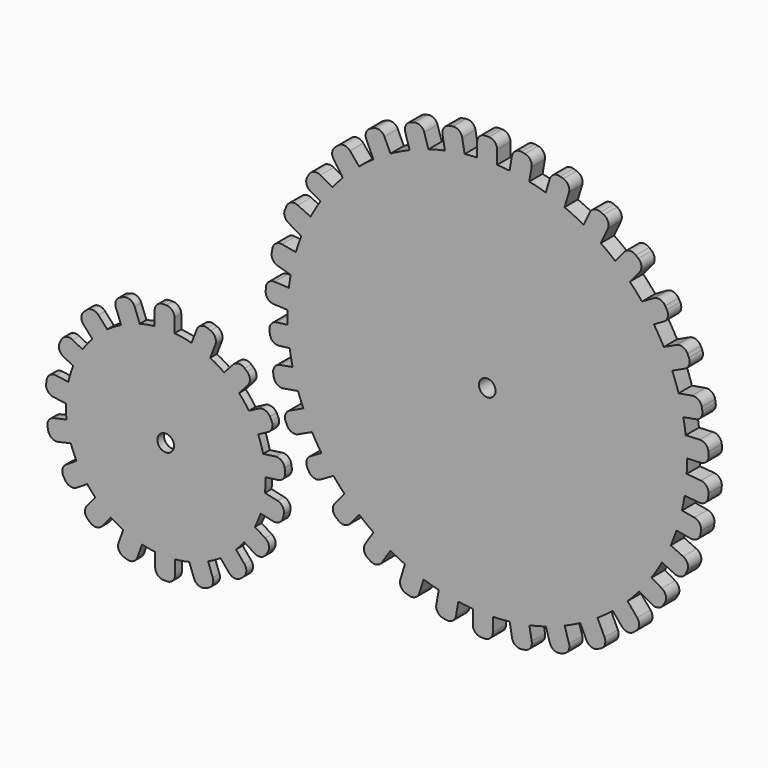
from build123d import *

# Parameters (mm, degrees)
F0_R     = 152.4
F0_R_2   = 6.35
F1_DEPTH = 12.7
F2_DEPTH = 6.35
F0_R_3   = 76.2
F4_DEPTH = 6.35
F6_DEPTH = 12.7


# Not quite as in the source:
# - a feature names something its author has since deleted; it is built from what else it names


with BuildPart() as f1:
    # F0 (on Front) → F1 (new body)
    with BuildSketch(Plane.XZ):
        with Locations((106.3798104379, 71.6841260691)):
            Circle(F0_R)
        with Locations((106.3798104379, 71.6841260691)):
            Circle(F0_R_2, mode=Mode.SUBTRACT)
    extrude(amount=F1_DEPTH)



with BuildPart() as f2:
    # F0 (on Front) → F2 (new body)
    with BuildSketch(Plane.XZ):
        with Locations((106.3798104379, 71.6841260691)):
            Circle(F0_R)
        with Locations((106.3798104379, 71.6841260691)):
            Circle(F0_R_2, mode=Mode.SUBTRACT)
    extrude(amount=F2_DEPTH)


with BuildPart() as f2b:
    # F0 (on Front) → F2, piece 2 (new body)
    with BuildSketch(Plane.XZ):
        with Locations((-144.0049031971, -49.3225429525)):
            Circle(F0_R_3)
        with Locations((-144.0049031971, -49.3225429525)):
            Circle(F0_R_2, mode=Mode.SUBTRACT)
    extrude(amount=F2_DEPTH)

    # F3 (on Front) → F4 (join)
    with BuildSketch(Plane.XZ):
        with BuildLine():
            Line((-204.3541227961, 20.4043868609), (-206.2390357075, 18.7018289862))
            ThreePointArc((-206.2390357075, 18.7018289862), (-208.3244533212, 14.3119079154), (-206.6949232994, 9.7331520212))
            Line((-206.6949232994, 9.7331520212), (-197.7369862783, -0.1842383959))
            ThreePointArc((-197.7369862783, -0.1842383959), (-197.2368223063, 0.0633153872), (-196.7901747778, 0.3979089611))
            Line((-196.7901747778, 0.3979089611), (-186.8162867746, 9.4068777351))
            ThreePointArc((-186.8162867746, 9.4068777351), (-186.5669051491, 9.6622880356), (-186.3514432182, 9.9468961399))
            Line((-186.3514432182, 9.9468961399), (-195.385445831, 19.948499269))
            ThreePointArc((-195.385445831, 19.948499269), (-199.7753669018, 22.0339168827), (-204.3541227961, 20.4043868609))
        make_face()
        with BuildLine():
            Line((-175.9440643065, 38.2304394299), (-178.3166684336, 37.3236044635))
            ThreePointArc((-178.3166684336, 37.3236044635), (-181.8468650713, 33.9832324288), (-181.9810913353, 29.1250067299))
            Line((-181.9810913353, 29.1250067299), (-176.9224404874, 15.8897695325))
            ThreePointArc((-176.9224404874, 15.8897695325), (-176.1952999555, 15.8943770065), (-175.4899473838, 16.0711037211))
            Line((-175.4899473838, 16.0711037211), (-164.0824814241, 20.4311606274))
            ThreePointArc((-164.0824814241, 20.4311606274), (-163.3354211249, 20.8437992565), (-162.7309690679, 21.446300244))
            Line((-162.7309690679, 21.446300244), (-167.7454665729, 34.5660165282))
            ThreePointArc((-167.7454665729, 34.5660165282), (-171.0858386076, 38.0962131659), (-175.9440643065, 38.2304394299))
        make_face()
        with BuildLine():
            Line((-143.5588021765, 43.2886108524), (-146.0988021765, 43.2886108524))
            ThreePointArc((-146.0988021765, 43.2886108524), (-150.588930237, 41.4287389129), (-152.4488021765, 36.9386108524))
            Line((-152.4488021765, 36.9386108524), (-152.4488021765, 23.5057070002))
            ThreePointArc((-152.4488021765, 23.5057070002), (-151.6256232188, 23.1059804274), (-150.7208942376, 22.9686108524))
            Line((-150.7208942376, 22.9686108524), (-138.5009451281, 22.9686108524))
            ThreePointArc((-138.5009451281, 22.9686108524), (-137.839627668, 23.0400251748), (-137.2088021765, 23.2509753769))
            Line((-137.2088021765, 23.2509753769), (-137.2088021765, 36.9386108524))
            ThreePointArc((-137.2088021765, 36.9386108524), (-139.068674116, 41.4287389129), (-143.5588021765, 43.2886108524))
        make_face()
        with BuildLine():
            ThreePointArc((-136.7876924353, -121.9389588268), (-137.3979774133, -121.7366523901), (-138.0371213199, -121.6668618795))
            Line((-138.0371213199, -121.6668618795), (-150.2997844964, -121.6668618795))
            ThreePointArc((-150.2997844964, -121.6668618795), (-151.2045134775, -121.8042314545), (-152.0276924353, -122.2039580274))
            Line((-152.0276924353, -122.2039580274), (-152.0276924353, -135.6368618795))
            ThreePointArc((-152.0276924353, -135.6368618795), (-150.1678204958, -140.12698994), (-145.6776924353, -141.9868618795))
            Line((-145.6776924353, -141.9868618795), (-143.1376924353, -141.9868618795))
            ThreePointArc((-143.1376924353, -141.9868618795), (-138.6475643747, -140.12698994), (-136.7876924353, -135.6368618795))
            Line((-136.7876924353, -135.6368618795), (-136.7876924353, -121.9389588268))
        make_face()
        with BuildLine():
            Line((-176.1923408536, -136.209608787), (-173.8052031826, -137.0774646159))
            ThreePointArc((-173.8052031826, -137.0774646159), (-168.9498273777, -136.8636903798), (-165.6677194328, -133.2792600109))
            Line((-165.6677194328, -133.2792600109), (-161.0693512083, -120.6309172247))
            ThreePointArc((-161.0693512083, -120.6309172247), (-161.7072488958, -119.9716351287), (-162.5124216468, -119.5320180423))
            Line((-162.5124216468, -119.5320180423), (-174.0098497748, -115.352070593))
            ThreePointArc((-174.0098497748, -115.352070593), (-174.6466853985, -115.1950207291), (-175.3023439103, -115.1766853205))
            Line((-175.3023439103, -115.1766853205), (-179.9905454586, -128.0721250372))
            ThreePointArc((-179.9905454586, -128.0721250372), (-179.7767712225, -132.9275008421), (-176.1923408536, -136.209608787))
        make_face()
        with BuildLine():
            Line((-203.3549844428, -120.0477373129), (-201.4090389886, -121.6801883196))
            ThreePointArc((-201.4090389886, -121.6801883196), (-196.7737263477, -123.1410956924), (-192.4630478364, -120.896452201))
            Line((-192.4630478364, -120.896452201), (-183.9812839196, -110.7858578437))
            ThreePointArc((-183.9812839196, -110.7858578437), (-184.3549387066, -109.9422037243), (-184.9639288475, -109.249021799))
            Line((-184.9639288475, -109.249021799), (-194.2361061545, -101.4706048106))
            ThreePointArc((-194.2361061545, -101.4706048106), (-194.8375854554, -101.0724913905), (-195.513143576, -100.8197210002))
            Line((-195.513143576, -100.8197210002), (-204.1387205614, -111.1017461607))
            ThreePointArc((-204.1387205614, -111.1017461607), (-205.5996279342, -115.7370588016), (-203.3549844428, -120.0477373129))
        make_face()
        with BuildLine():
            Line((-221.9770111308, -97.3072408044), (-220.6216536657, -99.455404239))
            ThreePointArc((-220.6216536657, -99.455404239), (-216.6527412723, -102.2604190419), (-211.8628514165, -101.437419163))
            Line((-211.8628514165, -101.437419163), (-201.5058619351, -94.902803229))
            ThreePointArc((-201.5058619351, -94.902803229), (-201.5923544651, -93.9512185842), (-201.9692402688, -93.0731802109))
            Line((-201.9692402688, -93.0731802109), (-208.5151537797, -82.6982847217))
            ThreePointArc((-208.5151537797, -82.6982847217), (-208.8884745428, -82.2224930782), (-209.3507880128, -81.8326054847))
            Line((-209.3507880128, -81.8326054847), (-219.9949962067, -88.5484385551))
            ThreePointArc((-219.9949962067, -88.5484385551), (-222.8000110096, -92.5173509486), (-221.9770111308, -97.3072408044))
        make_face()
        with BuildLine():
            Line((-234.1612291966, -67.9485382148), (-233.6126396119, -70.4285885101))
            ThreePointArc((-233.6126396119, -70.4285885101), (-230.8268862889, -74.4110440409), (-226.0410399119, -75.257240287))
            Line((-226.0410399119, -75.257240287), (-213.5840996431, -72.5017527468))
            ThreePointArc((-213.5840996431, -72.5017527468), (-213.3631563857, -71.6009829094), (-213.4233554896, -70.6754677605))
            Line((-213.4233554896, -70.6754677605), (-216.0944299344, -58.6001401358))
            ThreePointArc((-216.0944299344, -58.6001401358), (-216.2739099505, -58.0526065333), (-216.5576524317, -57.5511124393))
            Line((-216.5576524317, -57.5511124393), (-229.3325774197, -60.3769385147))
            ThreePointArc((-229.3325774197, -60.3769385147), (-233.3150329505, -63.1626918378), (-234.1612291966, -67.9485382148))
        make_face()
        with BuildLine():
            Line((-234.8751289908, -36.6048873101), (-235.2255460205, -39.1205995164))
            ThreePointArc((-235.2255460205, -39.1205995164), (-234.002914051, -43.8243793474), (-229.8123080788, -46.2859226067))
            Line((-229.8123080788, -46.2859226067), (-217.3849709244, -48.0169435724))
            ThreePointArc((-217.3849709244, -48.0169435724), (-216.82360206, -47.2265512804), (-216.5388459922, -46.2998534014))
            Line((-216.5388459922, -46.2998534014), (-214.8767964914, -34.3676758463))
            ThreePointArc((-214.8767964914, -34.3676758463), (-214.85853174, -33.6579630312), (-214.9993070039, -32.9621123245))
            Line((-214.9993070039, -32.9621123245), (-227.7098059006, -31.1916493684))
            ThreePointArc((-227.7098059006, -31.1916493684), (-232.4135857316, -32.4142813379), (-234.8751289908, -36.6048873101))
        make_face()
        with BuildLine():
            Line((-223.6030855792, -5.7841174114), (-224.7931154321, -8.0280935586))
            ThreePointArc((-224.7931154321, -8.0280935586), (-225.2536973874, -12.8662996202), (-222.1582496963, -16.6131085589))
            Line((-222.1582496963, -16.6131085589), (-212.1649924882, -21.9127524166))
            ThreePointArc((-212.1649924882, -21.9127524166), (-211.3178403266, -21.3555585105), (-210.7003788408, -20.5512742651))
            Line((-210.7003788408, -20.5512742651), (-204.9780904375, -9.7610586642))
            ThreePointArc((-204.9780904375, -9.7610586642), (-204.7580002749, -9.2207880669), (-204.6505108486, -8.6473963847))
            Line((-204.6505108486, -8.6473963847), (-215.0180705789, -3.1492516757))
            ThreePointArc((-215.0180705789, -3.1492516757), (-219.8562766405, -2.6886697204), (-223.6030855792, -5.7841174114))
        make_face()
        with BuildLine():
            Line((-114.0931942582, -115.352070593), (-125.5906223862, -119.5320180423))
            ThreePointArc((-125.5906223862, -119.5320180423), (-126.3957951373, -119.9716351287), (-127.0336928247, -120.6309172247))
            Line((-127.0336928247, -120.6309172247), (-122.4353246002, -133.2792600109))
            ThreePointArc((-122.4353246002, -133.2792600109), (-119.1532166553, -136.8636903798), (-114.2978408504, -137.0774646159))
            Line((-114.2978408504, -137.0774646159), (-111.9107031794, -136.209608787))
            ThreePointArc((-111.9107031794, -136.209608787), (-108.3262728106, -132.9275008421), (-108.1124985744, -128.0721250372))
            Line((-108.1124985744, -128.0721250372), (-112.8007001228, -115.1766853205))
            ThreePointArc((-112.8007001228, -115.1766853205), (-113.4563586346, -115.1950207291), (-114.0931942582, -115.352070593))
        make_face()
        with BuildLine():
            Line((-93.8669378785, -101.4706048106), (-103.1391151855, -109.249021799))
            ThreePointArc((-103.1391151855, -109.249021799), (-103.7481053264, -109.9422037243), (-104.1217601134, -110.7858578437))
            Line((-104.1217601134, -110.7858578437), (-95.6399961967, -120.896452201))
            ThreePointArc((-95.6399961967, -120.896452201), (-91.3293176854, -123.1410956924), (-86.6940050444, -121.6801883196))
            Line((-86.6940050444, -121.6801883196), (-84.7480595902, -120.0477373129))
            ThreePointArc((-84.7480595902, -120.0477373129), (-82.5034160989, -115.7370588016), (-83.9643234716, -111.1017461607))
            Line((-83.9643234716, -111.1017461607), (-92.589900457, -100.8197210002))
            ThreePointArc((-92.589900457, -100.8197210002), (-93.2654585777, -101.0724913905), (-93.8669378785, -101.4706048106))
        make_face()
        with BuildLine():
            Line((-79.5878902534, -82.6982847217), (-86.1338037642, -93.0731802109))
            ThreePointArc((-86.1338037642, -93.0731802109), (-86.5106895679, -93.9512185842), (-86.5971820979, -94.902803229))
            Line((-86.5971820979, -94.902803229), (-76.2401926166, -101.437419163))
            ThreePointArc((-76.2401926166, -101.437419163), (-71.4503027608, -102.2604190419), (-67.4813903673, -99.455404239))
            Line((-67.4813903673, -99.455404239), (-66.1260329023, -97.3072408044))
            ThreePointArc((-66.1260329023, -97.3072408044), (-65.3030330234, -92.5173509486), (-68.1080478263, -88.5484385551))
            Line((-68.1080478263, -88.5484385551), (-78.7522560203, -81.8326054847))
            ThreePointArc((-78.7522560203, -81.8326054847), (-79.2145694903, -82.2224930782), (-79.5878902534, -82.6982847217))
        make_face()
        with BuildLine():
            ThreePointArc((-71.5453916014, -57.5511124393), (-71.8291340826, -58.0526065333), (-72.0086140986, -58.6001401358))
            Line((-72.0086140986, -58.6001401358), (-74.6796885435, -70.6754677605))
            ThreePointArc((-74.6796885435, -70.6754677605), (-74.7398876473, -71.6009829094), (-74.51894439, -72.5017527468))
            Line((-74.51894439, -72.5017527468), (-62.0620041212, -75.257240287))
            ThreePointArc((-62.0620041212, -75.257240287), (-57.2761577442, -74.4110440409), (-54.4904044211, -70.4285885101))
            Line((-54.4904044211, -70.4285885101), (-53.9418148365, -67.9485382148))
            ThreePointArc((-53.9418148365, -67.9485382148), (-54.7880110826, -63.1626918378), (-58.7704666133, -60.3769385147))
            Line((-58.7704666133, -60.3769385147), (-71.5453916014, -57.5511124393))
        make_face()
        with BuildLine():
            Line((-73.2262475416, -34.3676758463), (-71.5641980408, -46.2998534014))
            ThreePointArc((-71.5641980408, -46.2998534014), (-71.2794419731, -47.2265512804), (-70.7180731086, -48.0169435724))
            Line((-70.7180731086, -48.0169435724), (-58.2907359542, -46.2859226067))
            ThreePointArc((-58.2907359542, -46.2859226067), (-54.100129982, -43.8243793474), (-52.8774980126, -39.1205995164))
            Line((-52.8774980126, -39.1205995164), (-53.2279150423, -36.6048873101))
            ThreePointArc((-53.2279150423, -36.6048873101), (-55.6894583015, -32.4142813379), (-60.3932381325, -31.1916493684))
            Line((-60.3932381325, -31.1916493684), (-73.1037370291, -32.9621123245))
            ThreePointArc((-73.1037370291, -32.9621123245), (-73.2445122931, -33.6579630312), (-73.2262475416, -34.3676758463))
        make_face()
        with BuildLine():
            Line((-83.1249535955, -9.7610586642), (-77.4026651923, -20.5512742651))
            ThreePointArc((-77.4026651923, -20.5512742651), (-76.7852037064, -21.3555585105), (-75.9380515448, -21.9127524166))
            Line((-75.9380515448, -21.9127524166), (-65.9447943367, -16.6131085589))
            ThreePointArc((-65.9447943367, -16.6131085589), (-62.8493466457, -12.8662996202), (-63.309928601, -8.0280935586))
            Line((-63.309928601, -8.0280935586), (-64.4999584539, -5.7841174114))
            ThreePointArc((-64.4999584539, -5.7841174114), (-68.2467673926, -2.6886697204), (-73.0849734541, -3.1492516757))
            Line((-73.0849734541, -3.1492516757), (-83.4525331844, -8.6473963847))
            ThreePointArc((-83.4525331844, -8.6473963847), (-83.3450437581, -9.2207880669), (-83.1249535955, -9.7610586642))
        make_face()
        with BuildLine():
            ThreePointArc((-101.7516008148, 9.9468961399), (-101.5361388839, 9.6622880356), (-101.2867572584, 9.4068777351))
            Line((-101.2867572584, 9.4068777351), (-91.3128692552, 0.3979089611))
            ThreePointArc((-91.3128692552, 0.3979089611), (-90.8662217267, 0.0633153872), (-90.3660577547, -0.1842383959))
            Line((-90.3660577547, -0.1842383959), (-81.4081207337, 9.7331520212))
            ThreePointArc((-81.4081207337, 9.7331520212), (-79.7785907119, 14.3119079154), (-81.8640083256, 18.7018289862))
            Line((-81.8640083256, 18.7018289862), (-83.748921237, 20.4043868609))
            ThreePointArc((-83.748921237, 20.4043868609), (-88.3276771312, 22.0339168827), (-92.717598202, 19.948499269))
            Line((-92.717598202, 19.948499269), (-101.7516008148, 9.9468961399))
        make_face()
        with BuildLine():
            Line((-124.0205626089, 20.4311606274), (-112.6130966493, 16.0711037211))
            ThreePointArc((-112.6130966493, 16.0711037211), (-111.9077440776, 15.8943770065), (-111.1806035456, 15.8897695325))
            Line((-111.1806035456, 15.8897695325), (-106.1219526978, 29.1250067299))
            ThreePointArc((-106.1219526978, 29.1250067299), (-106.2561789618, 33.9832324288), (-109.7863755995, 37.3236044635))
            Line((-109.7863755995, 37.3236044635), (-112.1589797265, 38.2304394299))
            ThreePointArc((-112.1589797265, 38.2304394299), (-117.0172054254, 38.0962131659), (-120.3575774601, 34.5660165282))
            Line((-120.3575774601, 34.5660165282), (-125.3720749651, 21.446300244))
            ThreePointArc((-125.3720749651, 21.446300244), (-124.7676229082, 20.8437992565), (-124.0205626089, 20.4311606274))
        make_face()
    extrude(amount=F4_DEPTH)


with BuildPart() as f1_1:
    add(f1.part)

    add(f2.part)  # F6 merges F2
    # F5 (on Front) → F6 (join)
    with BuildSketch(Plane.XZ):
        with BuildLine():
            ThreePointArc((-1.0245592963, 176.3703184272), (-0.8688153261, 176.4703400406), (-0.7221504189, 176.5832555508))
            Line((-0.7221504189, 176.5832555508), (9.3414453239, 185.0377039154))
            ThreePointArc((9.3414453239, 185.0377039154), (9.9458045347, 185.7248391814), (10.3189656625, 186.5603963023))
            Line((10.3189656625, 186.5603963023), (1.6784122703, 196.8455187117))
            ThreePointArc((1.6784122703, 196.8455187117), (-2.6338498025, 199.0871184635), (-7.2681299416, 197.6229390948))
            Line((-7.2681299416, 197.6229390948), (-9.674904736, 195.6010024287))
            ThreePointArc((-9.674904736, 195.6010024287), (-11.6445782491, 192.6544180871), (-11.7281303758, 189.1111156624))
            Line((-11.7281303758, 189.1111156624), (-1.0245592963, 176.3703184272))
        make_face()
        with BuildLine():
            ThreePointArc((-3.9138862135, 177.021707564), (-2.5974272967, 176.1273439582), (-1.0245592963, 176.3703184272))
            Line((-1.0245592963, 176.3703184272), (-11.7281303758, 189.1111156624))
            ThreePointArc((-11.7281303758, 189.1111156624), (-11.3645228576, 188.0967954669), (-10.8346522218, 187.1585561608))
            Line((-10.8346522218, 187.1585561608), (-3.9138862135, 177.021707564))
        make_face()
        with BuildLine():
            ThreePointArc((47.8904068269, 209.8163499975), (48.12467512, 209.8475296096), (48.3540937879, 209.9042823727))
            Line((48.3540937879, 209.9042823727), (60.8237512144, 213.7288847809))
            ThreePointArc((60.8237512144, 213.7288847809), (61.6484290935, 214.1255096984), (62.3182107431, 214.7490459615))
            Line((62.3182107431, 214.7490459615), (58.3792777757, 227.5914644634))
            ThreePointArc((58.3792777757, 227.5914644634), (55.2845212205, 231.3388442807), (50.4464001936, 231.8003186148))
            Line((50.4464001936, 231.8003186148), (48.0180538469, 231.0555139287))
            ThreePointArc((48.0180538469, 231.0555139287), (44.2706740297, 227.9607573735), (43.8091996955, 223.1226363466))
            Line((43.8091996955, 223.1226363466), (47.8904068269, 209.8163499975))
        make_face()
        with BuildLine():
            Line((20.0982469166, 195.7489624087), (32.341001256, 201.4666191011))
            ThreePointArc((32.341001256, 201.4666191011), (33.1026111195, 201.9739211269), (33.6793151863, 202.6844261225))
            Line((33.6793151863, 202.6844261225), (27.9951670721, 214.8554312624))
            ThreePointArc((27.9951670721, 214.8554312624), (24.4100104736, 218.1367459068), (19.5546820949, 217.9218972006))
            Line((19.5546820949, 217.9218972006), (17.2532919118, 216.8470933928))
            ThreePointArc((17.2532919118, 216.8470933928), (13.9719772675, 213.2619367943), (14.1868259737, 208.4066084156))
            Line((14.1868259737, 208.4066084156), (20.0982469166, 195.7489624087))
        make_face()
        with BuildLine():
            Line((76.0232179502, 217.3823675227), (88.0025690396, 219.5019140519))
            ThreePointArc((88.0025690396, 219.5019140519), (88.8695271021, 219.7948110427), (89.6104726789, 220.3318441718))
            Line((89.6104726789, 220.3318441718), (87.2700951432, 233.5592981555))
            ThreePointArc((87.2700951432, 233.5592981555), (84.6563665163, 237.6567115221), (79.9108725033, 238.7058350626))
            Line((79.9108725033, 238.7058350626), (77.4097205939, 238.2632979161))
            ThreePointArc((77.4097205939, 238.2632979161), (73.3123072273, 235.6495692892), (72.2631836868, 230.9040752762))
            Line((72.2631836868, 230.9040752762), (74.6444925558, 217.4452836898))
            ThreePointArc((74.6444925558, 217.4452836898), (75.3303693298, 217.3374361651), (76.0232179502, 217.3823675227))
        make_face()
        with BuildLine():
            Line((260.2206908891, 142.0700291107), (259.1472405042, 144.3720508898))
            ThreePointArc((259.1472405042, 144.3720508898), (255.5640139667, 147.6554730697), (250.7085600945, 147.4434793754))
            Line((250.7085600945, 147.4434793754), (238.5342147308, 141.7664888993))
            ThreePointArc((238.5342147308, 141.7664888993), (238.5198298854, 140.8515036504), (238.7776857592, 139.9734858386))
            Line((238.7776857592, 139.9734858386), (243.9968427597, 128.7809675318))
            ThreePointArc((243.9968427597, 128.7809675318), (244.3021755744, 128.2686537818), (244.7042014135, 127.8281214551))
            Line((244.7042014135, 127.8281214551), (257.1492624034, 133.6313487009))
            ThreePointArc((257.1492624034, 133.6313487009), (260.4326845834, 137.2145752385), (260.2206908891, 142.0700291107))
        make_face()
        with BuildLine():
            Line((243.4403321706, 168.7168144661), (242.1771492341, 170.9204407658))
            ThreePointArc((242.1771492341, 170.9204407658), (238.3305681834, 173.8909942245), (233.5101261434, 173.2715491737))
            Line((233.5101261434, 173.2715491737), (221.8561496827, 166.5911495934))
            ThreePointArc((221.8561496827, 166.5911495934), (221.9187392987, 165.6781942443), (222.2494979612, 164.8249629528))
            Line((222.2494979612, 164.8249629528), (227.2753059104, 156.057426396))
            ThreePointArc((227.2753059104, 156.057426396), (228.5033787541, 154.6410178722), (230.1757037272, 153.7938430378))
            Line((230.1757037272, 153.7938430378), (241.0892237627, 160.0497913754))
            ThreePointArc((241.0892237627, 160.0497913754), (244.0597772214, 163.8963724261), (243.4403321706, 168.7168144661))
        make_face()
        with BuildLine():
            Line((275.2757229067, 81.0317905346), (275.1540238465, 83.568873375))
            ThreePointArc((275.1540238465, 83.568873375), (273.0811523708, 87.9647325033), (268.507069095, 89.6073328251))
            Line((268.507069095, 89.6073328251), (255.0895927725, 88.9637218899))
            ThreePointArc((255.0895927725, 88.9637218899), (254.7297662673, 88.1223362377), (254.6359027536, 87.2120645364))
            Line((254.6359027536, 87.2120645364), (255.223383884, 74.9647366469))
            ThreePointArc((255.223383884, 74.9647366469), (255.3229520685, 74.3287374111), (255.5557510616, 73.7285595374))
            Line((255.5557510616, 73.7285595374), (269.2372634566, 74.3848357831))
            ThreePointArc((269.2372634566, 74.3848357831), (273.633122585, 76.4577072588), (275.2757229067, 81.0317905346))
        make_face()
        with BuildLine():
            Line((-42.592206737, 75.5533938816), (-42.0119272421, 87.8010650977))
            ThreePointArc((-42.0119272421, 87.8010650977), (-42.1063259871, 88.7112814492), (-42.4666471721, 89.5524553748))
            Line((-42.4666471721, 89.5524553748), (-55.8844996237, 90.1881766076))
            ThreePointArc((-55.8844996237, 90.1881766076), (-60.4576162457, 88.5428869696), (-62.5279025602, 84.1458097349))
            Line((-62.5279025602, 84.1458097349), (-62.6481097729, 81.6086557731))
            ThreePointArc((-62.6481097729, 81.6086557731), (-61.0028201349, 77.0355391511), (-56.6057429003, 74.9652528367))
            Line((-56.6057429003, 74.9652528367), (-42.9238469745, 74.3170215511))
            ThreePointArc((-42.9238469745, 74.3170215511), (-42.6914009313, 74.9173362088), (-42.592206737, 75.5533938816))
        make_face()
        with BuildLine():
            Line((270.5131564686, 109.6682831591), (270.0720900973, 112.1696948517))
            ThreePointArc((270.0720900973, 112.1696948517), (267.4607712365, 116.2686444048), (262.7158949375, 117.3205581552))
            Line((262.7158949375, 117.3205581552), (249.4870670785, 114.9879588805))
            ThreePointArc((249.4870670785, 114.9879588805), (249.2363567764, 114.1078740698), (249.2581786927, 113.1930359784))
            Line((249.2581786927, 113.1930359784), (251.2121747594, 102.1113736095))
            ThreePointArc((251.2121747594, 102.1113736095), (251.5913543929, 100.9785648168), (252.2853940364, 100.0062778589))
            Line((252.2853940364, 100.0062778589), (265.3622931652, 102.3120879993))
            ThreePointArc((265.3622931652, 102.3120879993), (269.4612427182, 104.9234068601), (270.5131564686, 109.6682831591))
        make_face()
        with BuildLine():
            Line((-38.6289994987, 102.0261590536), (-36.6815198823, 113.1089684732))
            ThreePointArc((-36.6815198823, 113.1089684732), (-36.6602359024, 114.0238192379), (-36.9114636586, 114.9037564765))
            Line((-36.9114636586, 114.9037564765), (-50.1416608191, 117.2285766837))
            ThreePointArc((-50.1416608191, 117.2285766837), (-54.8859177635, 116.1738730872), (-57.4948259553, 112.0733887649))
            Line((-57.4948259553, 112.0733887649), (-58.0494006059, 108.9173890257))
            ThreePointArc((-58.0494006059, 108.9173890257), (-57.6906086949, 105.4589639964), (-55.564270848, 102.707941881))
            Line((-55.564270848, 102.707941881), (-39.7009807757, 99.9204326047))
            ThreePointArc((-39.7009807757, 99.9204326047), (-39.0075129654, 100.8931274958), (-38.6289994987, 102.0261590536))
        make_face()
        with BuildLine():
            Line((-31.4293506964, 128.6999910423), (-26.2167758949, 139.8955763233))
            ThreePointArc((-26.2167758949, 139.8955763233), (-25.9594363477, 140.7737456048), (-25.9743592098, 141.6887222371))
            Line((-25.9743592098, 141.6887222371), (-38.152040588, 147.3585531123))
            ThreePointArc((-38.152040588, 147.3585531123), (-43.0076182748, 147.5676917214), (-46.5889135125, 144.2821631411))
            Line((-46.5889135125, 144.2821631411), (-47.9254367671, 141.4115741048))
            ThreePointArc((-47.9254367671, 141.4115741048), (-48.46871671, 137.9353323342), (-47.0778609789, 134.7034705984))
            Line((-47.0778609789, 134.7034705984), (-32.1361489462, 127.7467291975))
            ThreePointArc((-32.1361489462, 127.7467291975), (-31.7343822134, 128.1874978426), (-31.4293506964, 128.6999910423))
        make_face()
        with BuildLine():
            Line((-59.7967524833, 56.3136117376), (-59.4702737563, 53.7946810834))
            ThreePointArc((-59.4702737563, 53.7946810834), (-57.0486911835, 49.5808572292), (-52.3567503031, 48.3135512655))
            Line((-52.3567503031, 48.3135512655), (-41.8407955625, 49.6765246811))
            ThreePointArc((-41.8407955625, 49.6765246811), (-41.3847741945, 50.6920760446), (-41.3238471288, 51.8036460841))
            Line((-41.3238471288, 51.8036460841), (-43.0201186457, 64.8911460272))
            Line((-43.0201186457, 64.8911460272), (-54.3156226654, 63.4271351908))
            ThreePointArc((-54.3156226654, 63.4271351908), (-58.5294465197, 61.0055526181), (-59.7967524833, 56.3136117376))
        make_face()
        with BuildLine():
            Line((274.9560192353, 53.0251019398), (275.1773948219, 55.555436473))
            ThreePointArc((275.1773948219, 55.555436473), (273.7159407028, 60.190576761), (269.4049974554, 62.4347117723))
            Line((269.4049974554, 62.4347117723), (255.9048884791, 63.6158182641))
            ThreePointArc((255.9048884791, 63.6158182641), (255.4396240069, 62.8338566279), (255.2259104079, 61.9494011302))
            Line((255.2259104079, 61.9494011302), (254.3361911927, 51.7798639654))
            ThreePointArc((254.3361911927, 51.7798639654), (255.0985326357, 49.3620258071), (257.3472591972, 48.1914128535))
            Line((257.3472591972, 48.1914128535), (268.076743936, 47.2527045734))
            ThreePointArc((268.076743936, 47.2527045734), (272.7118842239, 48.7141586925), (274.9560192353, 53.0251019398))
        make_face()
        with BuildLine():
            Line((-14.7238555296, 155.9862775982), (-9.7032038361, 164.7567678576))
            ThreePointArc((-9.7032038361, 164.7567678576), (-9.372946938, 165.6101934904), (-9.3108941585, 166.5231854849))
            Line((-9.3108941585, 166.5231854849), (-20.9687967367, 173.1967312723))
            ThreePointArc((-20.9687967367, 173.1967312723), (-25.7896021823, 173.8133417547), (-29.6344358572, 170.8405269868))
            Line((-29.6344358572, 170.8405269868), (-30.8963228241, 168.6361583056))
            ThreePointArc((-30.8963228241, 168.6361583056), (-31.5129333066, 163.8153528601), (-28.5401185387, 159.9705191852))
            Line((-28.5401185387, 159.9705191852), (-17.6229218386, 153.7209891726))
            ThreePointArc((-17.6229218386, 153.7209891726), (-15.9510953007, 154.5691472019), (-14.7238555296, 155.9862775982))
        make_face()
        with BuildLine():
            ThreePointArc((-35.6241415015, 127.4124404853), (-33.8252209145, 127.0065006326), (-32.1361489462, 127.7467291975))
            Line((-32.1361489462, 127.7467291975), (-47.0778609789, 134.7034705984))
            ThreePointArc((-47.0778609789, 134.7034705984), (-46.3154336955, 133.9221774935), (-45.4304545802, 133.283016916))
            Line((-45.4304545802, 133.283016916), (-35.6241415015, 127.4124404853))
        make_face()
        with BuildLine():
            ThreePointArc((-43.7381548127, 98.8491770261), (-41.5702894989, 98.822229021), (-39.7009807757, 99.9204326047))
            Line((-39.7009807757, 99.9204326047), (-55.564270848, 102.707941881))
            ThreePointArc((-55.564270848, 102.707941881), (-54.6134250826, 102.1280363601), (-53.575886004, 101.7231774427))
            Line((-53.575886004, 101.7231774427), (-43.7381548127, 98.8491770261))
        make_face()
        with BuildLine():
            Line((251.6045288556, 99.8862229573), (252.2853940364, 100.0062778589))
            ThreePointArc((252.2853940364, 100.0062778589), (251.5913543929, 100.9785648168), (251.2121747594, 102.1113736095))
            Line((251.2121747594, 102.1113736095), (251.6045288556, 99.8862229573))
        make_face()
        with BuildLine():
            Line((-16.4160907922, 153.0301408668), (-14.7238555296, 155.9862775982))
            ThreePointArc((-14.7238555296, 155.9862775982), (-15.9510953007, 154.5691472019), (-17.6229218386, 153.7209891726))
            Line((-17.6229218386, 153.7209891726), (-16.4160907922, 153.0301408668))
        make_face()
        with BuildLine():
            ThreePointArc((203.1929267292, 185.0946970875), (202.5881635814, 185.7814768663), (202.2145112034, 186.6168144208))
            Line((202.2145112034, 186.6168144208), (201.8692724544, 186.2053749013))
            Line((201.8692724544, 186.2053749013), (203.1929267292, 185.0946970875))
        make_face()
        with BuildLine():
            ThreePointArc((10.3189656625, 186.5603963023), (9.9458045347, 185.7248391814), (9.3414453239, 185.0377039154))
            Line((9.3414453239, 185.0377039154), (10.6644462818, 186.1491598573))
            Line((10.6644462818, 186.1491598573), (10.3189656625, 186.5603963023))
        make_face()
        with BuildLine():
            Line((228.9692791142, 153.1022852244), (230.1757037272, 153.7938430378))
            ThreePointArc((230.1757037272, 153.7938430378), (228.5033787541, 154.6410178722), (227.2753059104, 156.057426396))
            Line((227.2753059104, 156.057426396), (228.9692791142, 153.1022852244))
        make_face()
        with BuildLine():
            Line((-42.0119272421, 87.8010650977), (-41.9301528337, 89.5270369375))
            Line((-41.9301528337, 89.5270369375), (-42.4666471721, 89.5524553748))
            ThreePointArc((-42.4666471721, 89.5524553748), (-42.1063259871, 88.7112814492), (-42.0119272421, 87.8010650977))
        make_face()
        with BuildLine():
            ThreePointArc((-41.3238471288, 51.8036460841), (-41.3847741945, 50.6920760446), (-41.8407955625, 49.6765246811))
            Line((-41.8407955625, 49.6765246811), (-41.0612462834, 49.7775621019))
            Line((-41.0612462834, 49.7775621019), (-41.3238471288, 51.8036460841))
        make_face()
        with BuildLine():
            Line((254.047499639, 48.4801044072), (257.3472591972, 48.1914128535))
            ThreePointArc((257.3472591972, 48.1914128535), (255.0985326357, 49.3620258071), (254.3361911927, 51.7798639654))
            Line((254.3361911927, 51.7798639654), (254.047499639, 48.4801044072))
        make_face()
        with BuildLine():
            Line((-39.0200451193, 99.8007780784), (-38.6289994987, 102.0261590536))
            ThreePointArc((-38.6289994987, 102.0261590536), (-39.0075129654, 100.8931274958), (-39.7009807757, 99.9204326047))
            Line((-39.7009807757, 99.9204326047), (-39.0200451193, 99.8007780784))
        make_face()
        with BuildLine():
            Line((-36.6815198823, 113.1089684732), (-36.3824724584, 114.8108017445))
            Line((-36.3824724584, 114.8108017445), (-36.9114636586, 114.9037564765))
            ThreePointArc((-36.9114636586, 114.9037564765), (-36.6602359024, 114.0238192379), (-36.6815198823, 113.1089684732))
        make_face()
        with BuildLine():
            Line((-26.2167758949, 139.8955763233), (-25.4874514027, 141.4620218635))
            Line((-25.4874514027, 141.4620218635), (-25.9743592098, 141.6887222371))
            ThreePointArc((-25.9743592098, 141.6887222371), (-25.9594363477, 140.7737456048), (-26.2167758949, 139.8955763233))
        make_face()
        with BuildLine():
            Line((-42.6513961102, 74.3041131665), (-42.592206737, 75.5533938816))
            ThreePointArc((-42.592206737, 75.5533938816), (-42.6914009313, 74.9173362088), (-42.9238469745, 74.3170215511))
            Line((-42.9238469745, 74.3170215511), (-42.6513961102, 74.3041131665))
        make_face()
        with BuildLine():
            ThreePointArc((249.2581786927, 113.1930359784), (249.2363567764, 114.1078740698), (249.4870670785, 114.9879588805))
            Line((249.4870670785, 114.9879588805), (248.9581306279, 114.8946931132))
            Line((248.9581306279, 114.8946931132), (249.2581786927, 113.1930359784))
        make_face()
        with BuildLine():
            ThreePointArc((255.2259104079, 61.9494011302), (255.4396240069, 62.8338566279), (255.9048884791, 63.6158182641))
            Line((255.9048884791, 63.6158182641), (255.3757531585, 63.6621116061))
            Line((255.3757531585, 63.6621116061), (255.2259104079, 61.9494011302))
        make_face()
        with BuildLine():
            ThreePointArc((254.6359027536, 87.2120645364), (254.7297662673, 88.1223362377), (255.0895927725, 88.9637218899))
            Line((255.0895927725, 88.9637218899), (254.5531134731, 88.9379879936))
            Line((254.5531134731, 88.9379879936), (254.6359027536, 87.2120645364))
        make_face()
        with BuildLine():
            ThreePointArc((222.2494979612, 164.8249629528), (221.9187392987, 165.6781942443), (221.8561496827, 166.5911495934))
            Line((221.8561496827, 166.5911495934), (221.3901814949, 166.3240430228))
            Line((221.3901814949, 166.3240430228), (222.2494979612, 164.8249629528))
        make_face()
        with BuildLine():
            Line((-9.7032038361, 164.7567678576), (-8.8447689903, 166.2563529538))
            Line((-8.8447689903, 166.2563529538), (-9.3108941585, 166.5231854849))
            ThreePointArc((-9.3108941585, 166.5231854849), (-9.372946938, 165.6101934904), (-9.7032038361, 164.7567678576))
        make_face()
        with BuildLine():
            ThreePointArc((238.7776857592, 139.9734858386), (238.5198298854, 140.8515036504), (238.5342147308, 141.7664888993))
            Line((238.5342147308, 141.7664888993), (238.0474403096, 141.5395022589))
            Line((238.0474403096, 141.5395022589), (238.7776857592, 139.9734858386))
        make_face()
        with BuildLine():
            Line((-31.9200309468, 127.6461063886), (-31.4293506964, 128.6999910423))
            ThreePointArc((-31.4293506964, 128.6999910423), (-31.7343822134, 128.1874978426), (-32.1361489462, 127.7467291975))
            Line((-32.1361489462, 127.7467291975), (-31.9200309468, 127.6461063886))
        make_face()
        with BuildLine():
            Line((255.2833078347, 73.7154909516), (255.5557510616, 73.7285595374))
            ThreePointArc((255.5557510616, 73.7285595374), (255.3229520685, 74.3287374111), (255.223383884, 74.9647366469))
            Line((255.223383884, 74.9647366469), (255.2833078347, 73.7154909516))
        make_face()
        with BuildLine():
            Line((213.5437897675, 176.4092917297), (213.5640260545, 176.4334083973))
            ThreePointArc((213.5640260545, 176.4334083973), (213.4082232976, 176.5333384147), (213.2614920205, 176.6461676651))
            Line((213.2614920205, 176.6461676651), (213.5437897675, 176.4092917297))
        make_face()
        with BuildLine():
            Line((-1.0245592963, 176.3703184272), (-1.0043088321, 176.3462136628))
            Line((-1.0043088321, 176.3462136628), (-0.7221504189, 176.5832555508))
            ThreePointArc((-0.7221504189, 176.5832555508), (-0.8688153261, 176.4703400406), (-1.0245592963, 176.3703184272))
        make_face()
        with BuildLine():
            Line((244.4881426185, 127.7273715844), (244.7042014135, 127.8281214551))
            ThreePointArc((244.7042014135, 127.8281214551), (244.3021755744, 128.2686537818), (243.9968427597, 128.7809675318))
            Line((243.9968427597, 128.7809675318), (244.4881426185, 127.7273715844))
        make_face()
        with BuildLine():
            Line((195.2623773151, 216.8994288321), (192.9603555361, 217.9728792169))
            ThreePointArc((192.9603555361, 217.9728792169), (188.1049016639, 218.1848729112), (184.5216751263, 214.9014507312))
            Line((184.5216751263, 214.9014507312), (178.8446846502, 202.7271053675))
            ThreePointArc((178.8446846502, 202.7271053675), (179.4218064004, 202.0169396017), (180.1837144301, 201.5100854968))
            Line((180.1837144301, 201.5100854968), (192.4298286842, 195.7996286374))
            Line((192.4298286842, 195.7996286374), (198.3338058008, 208.4607484223))
            ThreePointArc((198.3338058008, 208.4607484223), (198.5457994951, 213.3162022945), (195.2623773151, 216.8994288321))
        make_face()
        with BuildLine():
            Line((107.5767839528, 240.6254493239), (105.0367839528, 240.6254493239))
            ThreePointArc((105.0367839528, 240.6254493239), (100.5466558923, 238.7655773845), (98.6867839528, 234.2754493239))
            Line((98.6867839528, 234.2754493239), (98.6867839528, 220.8425454718))
            ThreePointArc((98.6867839528, 220.8425454718), (99.5099629106, 220.442818899), (100.4146918917, 220.3054493239))
            Line((100.4146918917, 220.3054493239), (112.3908374227, 220.3054493239))
            ThreePointArc((112.3908374227, 220.3054493239), (113.1816821157, 220.4012437289), (113.9267839528, 220.6830861469))
            Line((113.9267839528, 220.6830861469), (113.9267839528, 234.2754493239))
            ThreePointArc((113.9267839528, 234.2754493239), (112.0669120134, 238.7655773845), (107.5767839528, 240.6254493239))
        make_face()
        with BuildLine():
            Line((135.0933661208, 238.2802571568), (132.5919544281, 238.721323528))
            ThreePointArc((132.5919544281, 238.721323528), (127.8470781291, 237.6694097777), (125.2357592683, 233.5704602246))
            Line((125.2357592683, 233.5704602246), (122.9031599936, 220.3416323656))
            ThreePointArc((122.9031599936, 220.3416323656), (123.6444212224, 219.8050350117), (124.511551361, 219.5126478503))
            Line((124.511551361, 219.5126478503), (136.4921466909, 217.4001456486))
            ThreePointArc((136.4921466909, 217.4001456486), (137.1850216116, 217.3556216998), (137.8708348517, 217.4638725073))
            Line((137.8708348517, 217.4638725073), (140.2442294242, 230.924061997))
            ThreePointArc((140.2442294242, 230.924061997), (139.1923156738, 235.668938296), (135.0933661208, 238.2802571568))
        make_face()
        with BuildLine():
            Line((164.4892660254, 231.0897569677), (162.0604821469, 231.8331336366))
            ThreePointArc((162.0604821469, 231.8331336366), (157.2226333074, 231.3688145255), (154.1300807786, 227.6196156127))
            Line((154.1300807786, 227.6196156127), (150.1986999444, 214.7748832045))
            ThreePointArc((150.1986999444, 214.7748832045), (150.868848123, 214.1517408867), (151.6937590783, 213.7556009554))
            Line((151.6937590783, 213.7556009554), (164.1656632481, 209.9383314739))
            ThreePointArc((164.1656632481, 209.9383314739), (164.3951152475, 209.8817136208), (164.6294018339, 209.8506717658))
            Line((164.6294018339, 209.8506717658), (168.7027840493, 223.1593555994))
            ThreePointArc((168.7027840493, 223.1593555994), (168.2384649382, 227.9972044389), (164.4892660254, 231.0897569677))
        make_face()
        with BuildLine():
            Line((221.7408517825, 196.0570161353), (219.795098897, 197.689696664))
            ThreePointArc((219.795098897, 197.689696664), (215.1599586091, 199.151150783), (210.8490153617, 196.9070157717))
            Line((210.8490153617, 196.9070157717), (202.2145112034, 186.6168144208))
            ThreePointArc((202.2145112034, 186.6168144208), (202.5881635814, 185.7814768663), (203.1929267292, 185.0946970875))
            Line((203.1929267292, 185.0946970875), (213.2614920205, 176.6461676651))
            ThreePointArc((213.2614920205, 176.6461676651), (213.4082232976, 176.5333384147), (213.5640260545, 176.4334083973))
            Line((213.5640260545, 176.4334083973), (222.5235326748, 187.1109326))
            ThreePointArc((222.5235326748, 187.1109326), (223.9849867939, 191.746072888), (221.7408517825, 196.0570161353))
        make_face()
        with BuildLine():
            ThreePointArc((100.4146918917, 220.3054493239), (99.5099629106, 220.442818899), (98.6867839528, 220.8425454718))
            Line((98.6867839528, 220.8425454718), (98.6867839528, 220.3054493239))
            Line((98.6867839528, 220.3054493239), (100.4146918917, 220.3054493239))
        make_face()
        with BuildLine():
            Line((113.9267839528, 220.3054493239), (113.9267839528, 220.6830861469))
            ThreePointArc((113.9267839528, 220.6830861469), (113.1816821157, 220.4012437289), (112.3908374227, 220.3054493239))
            Line((112.3908374227, 220.3054493239), (113.9267839528, 220.3054493239))
        make_face()
        with BuildLine():
            ThreePointArc((151.6937590783, 213.7556009554), (150.868848123, 214.1517408867), (150.1986999444, 214.7748832045))
            Line((150.1986999444, 214.7748832045), (150.0415090998, 214.2613042812))
            Line((150.0415090998, 214.2613042812), (151.6937590783, 213.7556009554))
        make_face()
        with BuildLine():
            ThreePointArc((124.511551361, 219.5126478503), (123.6444212224, 219.8050350117), (122.9031599936, 220.3416323656))
            Line((122.9031599936, 220.3416323656), (122.8098942263, 219.812695915))
            Line((122.8098942263, 219.812695915), (124.511551361, 219.5126478503))
        make_face()
        with BuildLine():
            Line((137.8183643822, 217.1662976874), (137.8708348517, 217.4638725073))
            ThreePointArc((137.8708348517, 217.4638725073), (137.1850216116, 217.3556216998), (136.4921466909, 217.4001456486))
            Line((136.4921466909, 217.4001456486), (137.8183643822, 217.1662976874))
        make_face()
        with BuildLine():
            ThreePointArc((180.1837144301, 201.5100854968), (179.4218064004, 202.0169396017), (178.8446846502, 202.7271053675))
            Line((178.8446846502, 202.7271053675), (178.6176980098, 202.2403309463))
            Line((178.6176980098, 202.2403309463), (180.1837144301, 201.5100854968))
        make_face()
        with BuildLine():
            Line((164.6142123705, 209.801044268), (164.6294018339, 209.8506717658))
            ThreePointArc((164.6294018339, 209.8506717658), (164.3951152475, 209.8817136208), (164.1656632481, 209.9383314739))
            Line((164.1656632481, 209.9383314739), (164.6142123705, 209.801044268))
        make_face()
        with BuildLine():
            ThreePointArc((-35.8700178206, 23.0184345738), (-35.6193075185, 23.8985193844), (-35.6411294349, 24.8133574758))
            Line((-35.6411294349, 24.8133574758), (-37.5951255016, 35.8950198447))
            ThreePointArc((-37.5951255016, 35.8950198447), (-37.9743051351, 37.0278286374), (-38.6683447785, 38.0001155954))
            Line((-38.6683447785, 38.0001155954), (-51.7452439073, 35.694305455))
            ThreePointArc((-51.7452439073, 35.694305455), (-55.8441934604, 33.0829865942), (-56.8961072108, 28.3381102952))
            Line((-56.8961072108, 28.3381102952), (-56.4550408395, 25.8366986025))
            ThreePointArc((-56.4550408395, 25.8366986025), (-53.8437219787, 21.7377490495), (-49.0988456797, 20.6858352991))
            Line((-49.0988456797, 20.6858352991), (-35.8700178206, 23.0184345738))
        make_face()
        with BuildLine():
            ThreePointArc((-38.6683447785, 38.0001155954), (-37.9743051351, 37.0278286374), (-37.5951255016, 35.8950198447))
            Line((-37.5951255016, 35.8950198447), (-37.9874795977, 38.120170497))
            Line((-37.9874795977, 38.120170497), (-38.6683447785, 38.0001155954))
        make_face()
        with BuildLine():
            Line((-35.8700178206, 23.0184345738), (-35.3410813701, 23.1117003411))
            Line((-35.3410813701, 23.1117003411), (-35.6411294349, 24.8133574758))
            ThreePointArc((-35.6411294349, 24.8133574758), (-35.6193075185, 23.8985193844), (-35.8700178206, 23.0184345738))
        make_face()
        with BuildLine():
            ThreePointArc((-31.8491480295, 13.2262693971), (-31.4471221903, 12.7857370704), (-31.1417893757, 12.2734233205))
            Line((-31.1417893757, 12.2734233205), (-31.6330892345, 13.3270192678))
            Line((-31.6330892345, 13.3270192678), (-31.8491480295, 13.2262693971))
        make_face()
        with BuildLine():
            ThreePointArc((-17.5746538443, -11.8250636482), (-15.9023288712, -12.6722384825), (-14.6742560274, -14.0886470063))
            Line((-14.6742560274, -14.0886470063), (-16.3682292312, -11.1335058348))
            Line((-16.3682292312, -11.1335058348), (-17.5746538443, -11.8250636482))
        make_face()
        with BuildLine():
            Line((-25.6791613468, -0.7120980471), (-25.1923869256, -0.4851114067))
            Line((-25.1923869256, -0.4851114067), (-25.9226323752, 1.0809050137))
            ThreePointArc((-25.9226323752, 1.0809050137), (-25.6647765014, 0.2028872019), (-25.6791613468, -0.7120980471))
        make_face()
        with BuildLine():
            ThreePointArc((211.8475900346, -34.8079320352), (211.6918460643, -34.9079536486), (211.5451811572, -35.0208691588))
            Line((211.5451811572, -35.0208691588), (201.4815854143, -43.4753175234))
            ThreePointArc((201.4815854143, -43.4753175234), (200.8772262035, -44.1624527894), (200.5040650757, -44.9980099103))
            Line((200.5040650757, -44.9980099103), (209.144618468, -55.2831323197))
            ThreePointArc((209.144618468, -55.2831323197), (213.4568805407, -57.5247320715), (218.0911606798, -56.0605527028))
            Line((218.0911606798, -56.0605527028), (220.0359531988, -54.4267283371))
            ThreePointArc((220.0359531988, -54.4267283371), (222.2775529506, -50.1144662644), (220.8133735819, -45.4801861253))
            Line((220.8133735819, -45.4801861253), (211.8475900346, -34.8079320352))
        make_face()
        with BuildLine():
            ThreePointArc((137.9565573271, -74.104893323), (137.2706805531, -73.9970457983), (136.5778319327, -74.0419771558))
            Line((136.5778319327, -74.0419771558), (124.5984808434, -76.1615236851))
            ThreePointArc((124.5984808434, -76.1615236851), (123.7315227808, -76.4544206759), (122.990577204, -76.991453805))
            Line((122.990577204, -76.991453805), (125.3309547397, -90.2189077887))
            ThreePointArc((125.3309547397, -90.2189077887), (127.9446833666, -94.3163211553), (132.6901773797, -95.3654446958))
            Line((132.6901773797, -95.3654446958), (135.1913292891, -94.9229075493))
            ThreePointArc((135.1913292891, -94.9229075493), (139.2887426556, -92.3091789224), (140.3378661962, -87.5636849093))
            Line((140.3378661962, -87.5636849093), (137.9565573271, -74.104893323))
        make_face()
        with BuildLine():
            ThreePointArc((33.3354276297, -60.4100820146), (32.8611848642, -59.6274590346), (32.1760119267, -59.0208760022))
            Line((32.1760119267, -59.0208760022), (20.8290538751, -51.6844480673))
            Line((20.8290538751, -51.6844480673), (13.2440035523, -63.4159403679))
            ThreePointArc((13.2440035523, -63.4159403679), (12.3679281079, -68.1964074421), (15.1287499058, -72.1961870149))
            Line((15.1287499058, -72.1961870149), (17.2617485059, -73.5752870736))
            ThreePointArc((17.2617485059, -73.5752870736), (22.0422155801, -74.451362518), (26.041995153, -71.6905407201))
            Line((26.041995153, -71.6905407201), (33.3354276297, -60.4100820146))
        make_face()
        with BuildLine():
            ThreePointArc((164.710643056, -66.4759596307), (164.476374763, -66.5071392428), (164.246956095, -66.5638920059))
            Line((164.246956095, -66.5638920059), (151.7772986685, -70.3884944141))
            ThreePointArc((151.7772986685, -70.3884944141), (150.9526207894, -70.7851193316), (150.2828391398, -71.4086555946))
            Line((150.2828391398, -71.4086555946), (154.2217721072, -84.2510740966))
            ThreePointArc((154.2217721072, -84.2510740966), (157.3165286625, -87.9984539139), (162.1546496893, -88.459928248))
            Line((162.1546496893, -88.459928248), (164.582996036, -87.7151235619))
            ThreePointArc((164.582996036, -87.7151235619), (168.3303758533, -84.6203670067), (168.7918501874, -79.7822459798))
            Line((168.7918501874, -79.7822459798), (164.710643056, -66.4759596307))
        make_face()
        with BuildLine():
            Line((189.9627623606, -54.186558398), (177.7200080212, -59.9042150904))
            ThreePointArc((177.7200080212, -59.9042150904), (176.9583981577, -60.4115171162), (176.3816940909, -61.1220221118))
            Line((176.3816940909, -61.1220221118), (182.0658422051, -73.2930272517))
            ThreePointArc((182.0658422051, -73.2930272517), (185.6509988036, -76.5743418961), (190.5063271823, -76.3594931899))
            Line((190.5063271823, -76.3594931899), (192.8077173654, -75.2846893821))
            ThreePointArc((192.8077173654, -75.2846893821), (196.0890320097, -71.6995327836), (195.8741833035, -66.8442044049))
            Line((195.8741833035, -66.8442044049), (189.9627623606, -54.186558398))
        make_face()
        with BuildLine():
            Line((57.0972748545, -69.1452159143), (44.6253706847, -65.3279464328))
            ThreePointArc((44.6253706847, -65.3279464328), (44.3959186853, -65.2713285797), (44.1616320989, -65.2402867248))
            Line((44.1616320989, -65.2402867248), (40.0882498835, -78.5489705584))
            ThreePointArc((40.0882498835, -78.5489705584), (40.5525689946, -83.3868193979), (44.3017679074, -86.4793719267))
            Line((44.3017679074, -86.4793719267), (46.7305517859, -87.2227485955))
            ThreePointArc((46.7305517859, -87.2227485955), (51.5684006254, -86.7584294845), (54.6609531542, -83.0092305716))
            Line((54.6609531542, -83.0092305716), (58.5923339884, -70.1644981635))
            ThreePointArc((58.5923339884, -70.1644981635), (57.9221858098, -69.5413558456), (57.0972748545, -69.1452159143))
        make_face()
        with BuildLine():
            ThreePointArc((110.635225291, -77.4360033175), (109.8901234538, -77.1541608994), (109.0992787609, -77.0583664945))
            Line((109.0992787609, -77.0583664945), (97.1231332299, -77.0583664945))
            ThreePointArc((97.1231332299, -77.0583664945), (96.2184042487, -77.1957360695), (95.395225291, -77.5954626423))
            Line((95.395225291, -77.5954626423), (95.395225291, -91.0283664945))
            ThreePointArc((95.395225291, -91.0283664945), (97.2550972304, -95.518494555), (101.745225291, -97.3783664945))
            Line((101.745225291, -97.3783664945), (104.285225291, -97.3783664945))
            ThreePointArc((104.285225291, -97.3783664945), (108.7753533515, -95.518494555), (110.635225291, -91.0283664945))
            Line((110.635225291, -91.0283664945), (110.635225291, -77.4360033175))
        make_face()
        with BuildLine():
            ThreePointArc((84.8718900657, -75.9852592103), (84.130628837, -75.4486618564), (83.2634986983, -75.156274695))
            Line((83.2634986983, -75.156274695), (71.2829033684, -73.0437724934))
            ThreePointArc((71.2829033684, -73.0437724934), (70.5900284478, -72.9992485446), (69.9042152076, -73.1074993521))
            Line((69.9042152076, -73.1074993521), (67.5308206351, -86.5676888417))
            ThreePointArc((67.5308206351, -86.5676888417), (68.5827343855, -91.3125651408), (72.6816839386, -93.9238840016))
            Line((72.6816839386, -93.9238840016), (75.1830956312, -94.3649503728))
            ThreePointArc((75.1830956312, -94.3649503728), (79.9279719302, -93.3130366224), (82.539290791, -89.2140870694))
            Line((82.539290791, -89.2140870694), (84.8718900657, -75.9852592103))
        make_face()
        with BuildLine():
            ThreePointArc((95.395225291, -77.5954626423), (96.2184042487, -77.1957360695), (97.1231332299, -77.0583664945))
            Line((97.1231332299, -77.0583664945), (95.395225291, -77.0583664945))
            Line((95.395225291, -77.0583664945), (95.395225291, -77.5954626423))
        make_face()
        with BuildLine():
            Line((110.635225291, -77.4360033175), (110.635225291, -77.0583664945))
            Line((110.635225291, -77.0583664945), (109.0992787609, -77.0583664945))
            ThreePointArc((109.0992787609, -77.0583664945), (109.8901234538, -77.1541608994), (110.635225291, -77.4360033175))
        make_face()
        with BuildLine():
            Line((58.749524833, -69.6509192402), (57.0972748545, -69.1452159143))
            ThreePointArc((57.0972748545, -69.1452159143), (57.9221858098, -69.5413558456), (58.5923339884, -70.1644981635))
            Line((58.5923339884, -70.1644981635), (58.749524833, -69.6509192402))
        make_face()
        with BuildLine():
            Line((10.7317774286, -42.8649845345), (9.4081231537, -41.7543067207))
            ThreePointArc((9.4081231537, -41.7543067207), (10.0128863015, -42.4410864995), (10.3865386795, -43.276424054))
            Line((10.3865386795, -43.276424054), (10.7317774286, -42.8649845345))
        make_face()
        with BuildLine():
            Line((33.3354276297, -60.4100820146), (33.6270454758, -59.9590484195))
            Line((33.6270454758, -59.9590484195), (32.1760119267, -59.0208760022))
            ThreePointArc((32.1760119267, -59.0208760022), (32.8611848642, -59.6274590346), (33.3354276297, -60.4100820146))
        make_face()
        with BuildLine():
            Line((44.6253706847, -65.3279464328), (44.1768215623, -65.1906592269))
            Line((44.1768215623, -65.1906592269), (44.1616320989, -65.2402867248))
            ThreePointArc((44.1616320989, -65.2402867248), (44.3959186853, -65.2713285797), (44.6253706847, -65.3279464328))
        make_face()
        with BuildLine():
            ThreePointArc((150.2828391398, -71.4086555946), (150.9526207894, -70.7851193316), (151.7772986685, -70.3884944141))
            Line((151.7772986685, -70.3884944141), (150.1253463336, -70.8951691897))
            Line((150.1253463336, -70.8951691897), (150.2828391398, -71.4086555946))
        make_face()
        with BuildLine():
            ThreePointArc((200.5040650757, -44.9980099103), (200.8772262035, -44.1624527894), (201.4815854143, -43.4753175234))
            Line((201.4815854143, -43.4753175234), (200.1585844564, -44.5867734653))
            Line((200.1585844564, -44.5867734653), (200.5040650757, -44.9980099103))
        make_face()
        with BuildLine():
            Line((137.9565573271, -74.104893323), (137.9039118901, -73.8073494076))
            Line((137.9039118901, -73.8073494076), (136.5778319327, -74.0419771558))
            ThreePointArc((136.5778319327, -74.0419771558), (137.2706805531, -73.9970457983), (137.9565573271, -74.104893323))
        make_face()
        with BuildLine():
            Line((164.710643056, -66.4759596307), (164.6954244138, -66.426341073))
            Line((164.6954244138, -66.426341073), (164.246956095, -66.5638920059))
            ThreePointArc((164.246956095, -66.5638920059), (164.476374763, -66.5071392428), (164.710643056, -66.4759596307))
        make_face()
        with BuildLine():
            Line((177.7200080212, -59.9042150904), (176.1544212622, -60.6353812448))
            Line((176.1544212622, -60.6353812448), (176.3816940909, -61.1220221118))
            ThreePointArc((176.3816940909, -61.1220221118), (176.9583981577, -60.4115171162), (177.7200080212, -59.9042150904))
        make_face()
        with BuildLine():
            ThreePointArc((122.990577204, -76.991453805), (123.7315227808, -76.4544206759), (124.5984808434, -76.1615236851))
            Line((124.5984808434, -76.1615236851), (122.8970004337, -76.462572287))
            Line((122.8970004337, -76.462572287), (122.990577204, -76.991453805))
        make_face()
        with BuildLine():
            ThreePointArc((69.9042152076, -73.1074993521), (70.5900284478, -72.9992485446), (71.2829033684, -73.0437724934))
            Line((71.2829033684, -73.0437724934), (69.9566856771, -72.8099245322))
            Line((69.9566856771, -72.8099245322), (69.9042152076, -73.1074993521))
        make_face()
        with BuildLine():
            Line((84.8718900657, -75.9852592103), (84.9651558331, -75.4563227598))
            Line((84.9651558331, -75.4563227598), (83.2634986983, -75.156274695))
            ThreePointArc((83.2634986983, -75.156274695), (84.130628837, -75.4486618564), (84.8718900657, -75.9852592103))
        make_face()
        with BuildLine():
            Line((211.8475900346, -34.8079320352), (211.8273395703, -34.7838272708))
            Line((211.8273395703, -34.7838272708), (211.5451811572, -35.0208691588))
            ThreePointArc((211.5451811572, -35.0208691588), (211.6918460643, -34.9079536486), (211.8475900346, -34.8079320352))
        make_face()
        with BuildLine():
            Line((-0.6604421375, -33.3057772983), (-0.9427398846, -33.0689013629))
            Line((-0.9427398846, -33.0689013629), (-0.9629761715, -33.0930180305))
            ThreePointArc((-0.9629761715, -33.0930180305), (-0.8071734146, -33.1929480479), (-0.6604421375, -33.3057772983))
        make_face()
        with BuildLine():
            ThreePointArc((237.547823515, 0.6508140549), (237.2904839678, -0.2273552266), (237.3054068299, -1.1423318589))
            Line((237.3054068299, -1.1423318589), (249.483088208, -6.8121627341))
            ThreePointArc((249.483088208, -6.8121627341), (254.3386658949, -7.0213013432), (257.9199611326, -3.735772763))
            Line((257.9199611326, -3.735772763), (258.9920577233, -1.4331201838))
            ThreePointArc((258.9920577233, -1.4331201838), (259.2011963324, 3.4224575031), (255.9156677521, 7.0037527408))
            Line((255.9156677521, 7.0037527408), (243.4671965662, 12.7996611807))
            ThreePointArc((243.4671965662, 12.7996611807), (243.0654298334, 12.3588925356), (242.7603983164, 11.8463993358))
            Line((242.7603983164, 11.8463993358), (237.547823515, 0.6508140549))
        make_face()
        with BuildLine():
            Line((225.800887611, -15.6938861567), (220.7802359174, -24.464376416))
            ThreePointArc((220.7802359174, -24.464376416), (220.4499790193, -25.3178020489), (220.3879262398, -26.2307940434))
            Line((220.3879262398, -26.2307940434), (232.045828818, -32.9043398307))
            ThreePointArc((232.045828818, -32.9043398307), (236.8666342636, -33.5209503131), (240.7114679385, -30.5481355453))
            Line((240.7114679385, -30.5481355453), (241.9733549055, -28.3437668641))
            ThreePointArc((241.9733549055, -28.3437668641), (242.5899653879, -23.5229614185), (239.61715062, -19.6781277437))
            Line((239.61715062, -19.6781277437), (228.69995392, -13.4285977311))
            ThreePointArc((228.69995392, -13.4285977311), (227.028127382, -14.2767557604), (225.800887611, -15.6938861567))
        make_face()
        with BuildLine():
            ThreePointArc((248.2411668522, 25.0752128241), (248.2198828723, 24.1603620594), (248.4711106285, 23.2804248207))
            Line((248.4711106285, 23.2804248207), (261.7013077889, 20.9556046136))
            ThreePointArc((261.7013077889, 20.9556046136), (266.4455647334, 22.0103082101), (269.0544729252, 26.1107925324))
            Line((269.0544729252, 26.1107925324), (269.4940683687, 28.6124631434))
            ThreePointArc((269.4940683687, 28.6124631434), (268.4393647722, 33.3567200878), (264.3388804498, 35.9656282797))
            Line((264.3388804498, 35.9656282797), (251.2606277456, 38.2637486926))
            ThreePointArc((251.2606277456, 38.2637486926), (250.5671599352, 37.2910538015), (250.1886464686, 36.1580222437))
            Line((250.1886464686, 36.1580222437), (248.2411668522, 25.0752128241))
        make_face()
        with BuildLine():
            Line((227.4931228735, -12.7377494252), (225.800887611, -15.6938861567))
            ThreePointArc((225.800887611, -15.6938861567), (227.028127382, -14.2767557604), (228.69995392, -13.4285977311))
            Line((228.69995392, -13.4285977311), (227.4931228735, -12.7377494252))
        make_face()
        with BuildLine():
            Line((247.9421194283, 23.3733795527), (248.4711106285, 23.2804248207))
            ThreePointArc((248.4711106285, 23.2804248207), (248.2198828723, 24.1603620594), (248.2411668522, 25.0752128241))
            Line((248.2411668522, 25.0752128241), (247.9421194283, 23.3733795527))
        make_face()
        with BuildLine():
            Line((243.2510785669, 12.9002839895), (242.7603983164, 11.8463993358))
            ThreePointArc((242.7603983164, 11.8463993358), (243.0654298334, 12.3588925356), (243.4671965662, 12.7996611807))
            Line((243.4671965662, 12.7996611807), (243.2510785669, 12.9002839895))
        make_face()
        with BuildLine():
            Line((250.5796920892, 38.3834032189), (250.1886464686, 36.1580222437))
            ThreePointArc((250.1886464686, 36.1580222437), (250.5671599352, 37.2910538015), (251.2606277456, 38.2637486926))
            Line((251.2606277456, 38.2637486926), (250.5796920892, 38.3834032189))
        make_face()
        with BuildLine():
            Line((236.8184990227, -0.9156314853), (237.3054068299, -1.1423318589))
            ThreePointArc((237.3054068299, -1.1423318589), (237.2904839678, -0.2273552266), (237.547823515, 0.6508140549))
            Line((237.547823515, 0.6508140549), (236.8184990227, -0.9156314853))
        make_face()
        with BuildLine():
            Line((220.7802359174, -24.464376416), (219.9218010716, -25.9639615123))
            Line((219.9218010716, -25.9639615123), (220.3879262398, -26.2307940434))
            ThreePointArc((220.3879262398, -26.2307940434), (220.4499790193, -25.3178020489), (220.7802359174, -24.464376416))
        make_face()
        with BuildLine():
            ThreePointArc((-25.6791613468, -0.7120980471), (-25.6647765014, 0.2028872019), (-25.9226323752, 1.0809050137))
            Line((-25.9226323752, 1.0809050137), (-31.1417893757, 12.2734233205))
            ThreePointArc((-31.1417893757, 12.2734233205), (-31.4471221903, 12.7857370704), (-31.8491480295, 13.2262693971))
            Line((-31.8491480295, 13.2262693971), (-44.2942090194, 7.4230421513))
            ThreePointArc((-44.2942090194, 7.4230421513), (-47.5776311994, 3.8398156137), (-47.3656375051, -1.0156382585))
            Line((-47.3656375051, -1.0156382585), (-46.2921871202, -3.3176600375))
            ThreePointArc((-46.2921871202, -3.3176600375), (-42.7089605827, -6.6010822175), (-37.8535067105, -6.3890885232))
            Line((-37.8535067105, -6.3890885232), (-25.6791613468, -0.7120980471))
        make_face()
        with BuildLine():
            ThreePointArc((-9.2550997998, -24.6223702037), (-9.3176894158, -23.7094148546), (-9.6484480783, -22.8561835632))
            Line((-9.6484480783, -22.8561835632), (-14.6742560274, -14.0886470063))
            ThreePointArc((-14.6742560274, -14.0886470063), (-15.9023288712, -12.6722384825), (-17.5746538443, -11.8250636482))
            Line((-17.5746538443, -11.8250636482), (-28.4881738797, -18.0810119857))
            ThreePointArc((-28.4881738797, -18.0810119857), (-31.4587273385, -21.9275930364), (-30.8392822877, -26.7480350764))
            Line((-30.8392822877, -26.7480350764), (-29.5760993512, -28.9516613761))
            ThreePointArc((-29.5760993512, -28.9516613761), (-25.7295183004, -31.9222148349), (-20.9090762605, -31.3027697841))
            Line((-20.9090762605, -31.3027697841), (-9.2550997998, -24.6223702037))
        make_face()
        with BuildLine():
            Line((9.4081231537, -41.7543067207), (-0.6604421375, -33.3057772983))
            ThreePointArc((-0.6604421375, -33.3057772983), (-0.8071734146, -33.1929480479), (-0.9629761715, -33.0930180305))
            Line((-0.9629761715, -33.0930180305), (-9.9224827919, -43.7705422332))
            ThreePointArc((-9.9224827919, -43.7705422332), (-11.383936911, -48.4056825212), (-9.1398018996, -52.7166257685))
            Line((-9.1398018996, -52.7166257685), (-7.1940490141, -54.3493062971))
            ThreePointArc((-7.1940490141, -54.3493062971), (-2.5589087261, -55.8107604162), (1.7520345212, -53.5666254048))
            Line((1.7520345212, -53.5666254048), (10.3865386795, -43.276424054))
            ThreePointArc((10.3865386795, -43.276424054), (10.0128863015, -42.4410864995), (9.4081231537, -41.7543067207))
        make_face()
    extrude(amount=F6_DEPTH)


solid = Compound([f2b.part, f1_1.part])
